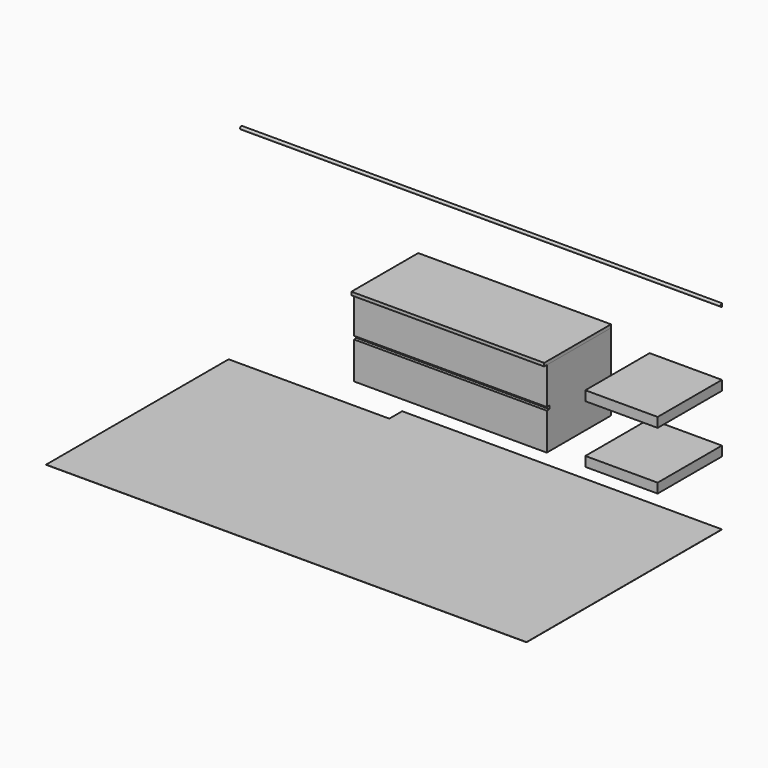
from build123d import *

# Parameters (mm, degrees)
F2_DEPTH  = 0.1
F3_W      = 120
F3_H      = 2
F4_DEPTH  = 48
F3_H_2    = 23
F5_DEPTH  = 50
F6_DEPTH  = 52
F8_DEPTH  = 299
F3_W_2    = 45
F3_H_3    = 6
F10_DEPTH = 50


# Not quite as in the source:
# - the program builds the solid bodies; features that only make, move or delete a surface that nothing else refers to are left out


with BuildPart() as f2:
    # F0 (on Top) → F2 (new body)
    with BuildSketch(Plane.XY):
        Polygon((0, -52), (0, 0), (-199, 0), (-199, -10), (-299, -10), (-299, -152), (0, -152), align=None)
    extrude(amount=F2_DEPTH)


with BuildPart() as f4:
    # F3 (on face) → F4 (new body)
    with BuildSketch(Plane(origin=(0, 0, 0), x_dir=(-1, 0, 0), z_dir=(0, 1, 0))):
        with Locations((129, 64)):
            Rectangle(F3_W, F3_H)
    extrude(amount=-F4_DEPTH)

    # F3 (on face) → F5 (join)
    with BuildSketch(Plane(origin=(0, 0, 0), x_dir=(-1, 0, 0), z_dir=(0, 1, 0))):
        with Locations((129, 76.5)):
            Rectangle(F3_W, F3_H_2)
        with Locations((129, 51.5)):
            Rectangle(F3_W, F3_H_2)
    extrude(amount=-F5_DEPTH)


with BuildPart() as f6:
    # F3 (on face) → F6 (new body)
    with BuildSketch(Plane(origin=(0, 0, 0), x_dir=(-1, 0, 0), z_dir=(0, 1, 0))):
        with Locations((129, 89)):
            Rectangle(F3_W, F3_H)
    extrude(amount=-F6_DEPTH)


with BuildPart() as f8:
    # F7 (on face) → F8 (new body)
    with BuildSketch(Plane.YZ):
        with BuildLine():
            ThreePointArc((0, 124), (-1, 123), (0, 122))
            Line((0, 122), (0, 124))
        make_face()
    extrude(amount=-F8_DEPTH)


with BuildPart() as f10:
    # F3 (on face) → F10 (new body)
    with BuildSketch(Plane(origin=(0, 0, 0), x_dir=(-1, 0, 0), z_dir=(0, 1, 0))):
        with Locations((22.5, 79)):
            Rectangle(F3_W_2, F3_H_3)
    extrude(amount=-F10_DEPTH)


with BuildPart() as f10b:
    # F3 (on face) → F10, piece 2 (new body)
    with BuildSketch(Plane(origin=(0, 0, 0), x_dir=(-1, 0, 0), z_dir=(0, 1, 0))):
        with Locations((22.5, 43)):
            Rectangle(F3_W_2, F3_H_3)
    extrude(amount=-F10_DEPTH)


solid = Compound([f2.part, f4.part, f6.part, f8.part, f10.part, f10b.part])
